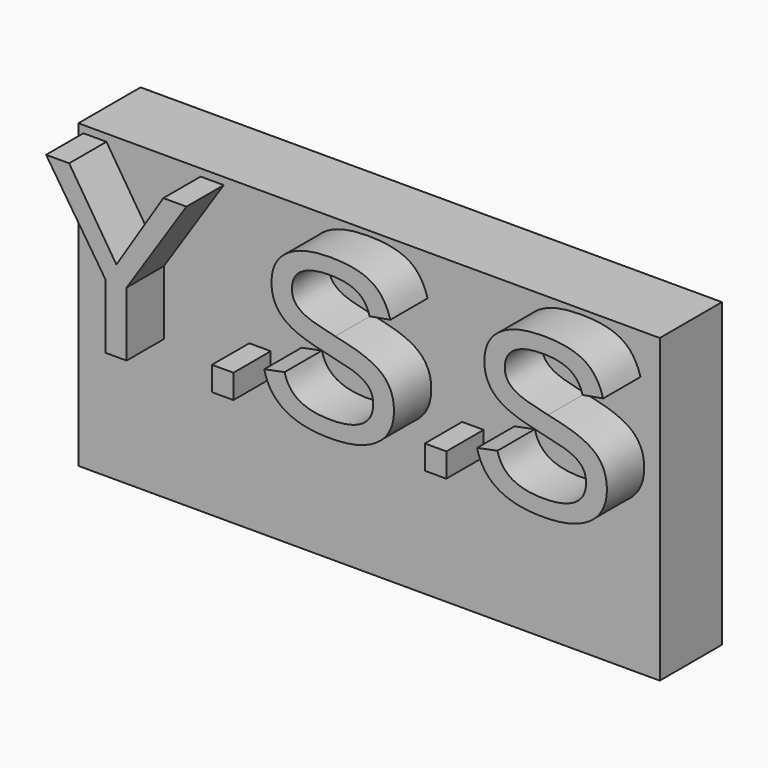
from build123d import *

# Parameters (mm, degrees)
F0_W         = 95.0349122286
F0_H         = 49.3149235845
F1_DEPTH     = 12.7
F2_TEXT_SIZE = 36.8330066168
F3_DEPTH     = 7.62


# Not quite as in the source:
# - Text() gives the source's letters only with a copy of the font that has no kerning and outlines rounded to 1/6400 em; it was checked with that copy


with BuildPart() as f1:
    # F0 (on Front) → F1 (new body)
    with BuildSketch(Plane.XZ):
        with Locations((47.5174561143, 24.6574617922)):
            Rectangle(F0_W, F0_H)
    extrude(amount=F1_DEPTH)

    # F2 (on face) → F3 (join)
    with BuildSketch(Plane.XZ.offset(12.7)):
        with Locations((0, 22.7951588204)):
            Text('Y.S.S', F2_TEXT_SIZE, font='Arimo', text_align=(TextAlign.LEFT, TextAlign.BOTTOM))
    extrude(amount=F3_DEPTH)


solid = f1.part
